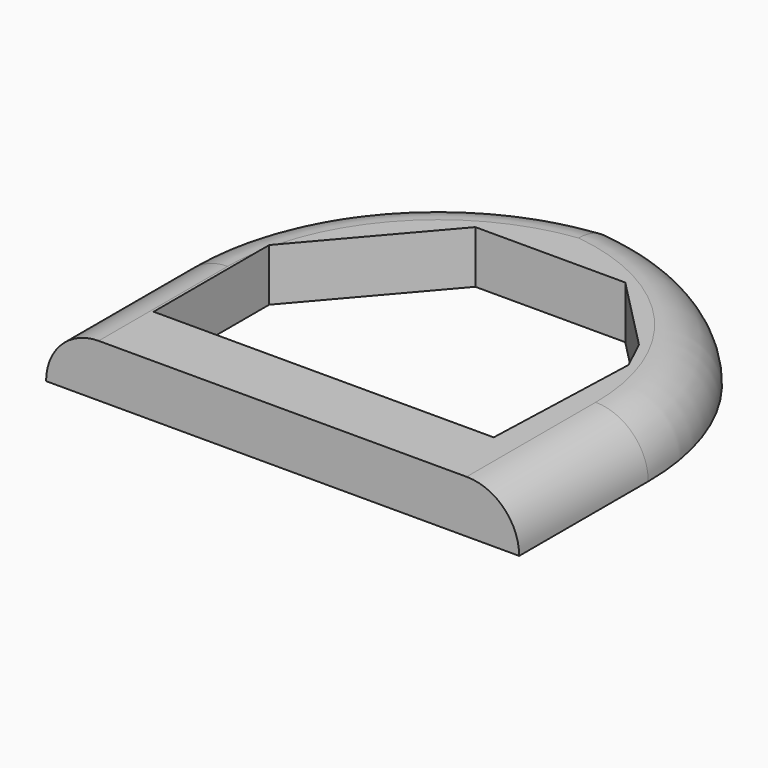
from build123d import *

# Parameters (mm, degrees)
F0_W        = 45.72
F0_H        = 40.9903422
F1_DEPTH    = 5.08
F2_T1_DEPTH = 132.08
F4_DEPTH    = 25.4
F5_T1_DEPTH = 28.2903422
F5_T4_ANGLE = 112.9188061074
F5_T6_ANGLE = 112.9188061074


# Not quite as in the source:
# - a fillet or chamfer that OpenCascade refuses, or shapes differently, is made with other operations: its cross-section is extruded or revolved along the edge and cut away or added


with BuildPart() as f1:
    # F0 (on Top) → F1 (new body)
    with BuildSketch(Plane.XY):
        with Locations((22.86, 20.4951711)):
            Rectangle(F0_W, F0_H)
    extrude(amount=F1_DEPTH)

    # F2: fillet of radius 25.4 on 2 edges, made by hand

    # F2_s2 → F2_t1 (cut)
    with BuildSketch(Plane.XY.offset(-63.5)):
        with BuildLine():
            ThreePointArc((25.4, 40.9903422), (7.4394877579, 33.5508544421), (0, 15.5903422))
            Line((0, 15.5903422), (0, 40.9903422))
            Line((0, 40.9903422), (25.4, 40.9903422))
        make_face()
        with BuildLine():
            ThreePointArc((20.32, 40.9903422), (38.2805122421, 33.5508544421), (45.72, 15.5903422))
            Line((45.72, 15.5903422), (45.72, 40.9903422))
            Line((45.72, 40.9903422), (20.32, 40.9903422))
        make_face()
    extrude(amount=F2_T1_DEPTH, mode=Mode.SUBTRACT)

    # F3 (on face) → F4 (cut)
    with BuildSketch(Plane.XY.offset(5.08)):
        Polygon((5.343540106, 6.3080484979), (38.2127352059, 6.3080484979), (38.763590157, 21.9034794718), (37.315774709, 24.9750651419), (30.1536079496, 32.2724170983), (22.2911257297, 32.2724170983), (15.6609918922, 32.2724170983), (5.343540106, 20.2690735459), align=None)
    extrude(amount=-F4_DEPTH, mode=Mode.SUBTRACT)

    # F5: fillet of radius 5.08 on 4 edges, made by hand

    # F5_s2 → F5_t1 (cut)
    with BuildSketch(Plane.XZ.offset(-15.5903422)):
        with BuildLine():
            ThreePointArc((45.72, 0), (44.2321024484, 3.5921024484), (40.64, 5.08))
            Line((40.64, 5.08), (45.72, 5.08))
            Line((45.72, 5.08), (45.72, 0))
        make_face()
        with BuildLine():
            ThreePointArc((5.08, 5.08), (1.4878975516, 3.5921024484), (0, 0))
            Line((0, 0), (0, 5.08))
            Line((0, 5.08), (5.08, 5.08))
        make_face()
    extrude(amount=F5_T1_DEPTH, mode=Mode.SUBTRACT)

    # F5_s3 → F5_t4 (revolve, cut)
    with BuildSketch(Plane(origin=(22.8304215849, 9.6527795985, 0), x_dir=(0, 0, 1), z_dir=(-0.9210576344, -0.3894262885, 0))):
        with BuildLine():
            ThreePointArc((0, 31.8464615241), (3.5921024484, 30.3585639725), (5.08, 26.7664615241))
            Line((5.08, 26.7664615241), (5.08, 31.8464615241))
            Line((5.08, 31.8464615241), (0, 31.8464615241))
        make_face()
    revolve(axis=Axis((20.3199999999, 15.5903421999, 5.08), (0, 0, -1)), revolution_arc=F5_T4_ANGLE, mode=Mode.SUBTRACT)

    # F5_s5 → F5_t6 (revolve, cut)
    with BuildSketch(Plane.XZ.offset(-15.5903421999)):
        with BuildLine():
            ThreePointArc((5.08, 5.08), (1.4878975516, 3.5921024484), (0, 0))
            Line((0, 0), (0, 5.08))
            Line((0, 5.08), (5.08, 5.08))
        make_face()
    revolve(axis=Axis((25.4000000001, 15.5903421999, 5.08), (0, 0, -1)), revolution_arc=F5_T6_ANGLE, mode=Mode.SUBTRACT)


solid = f1.part
